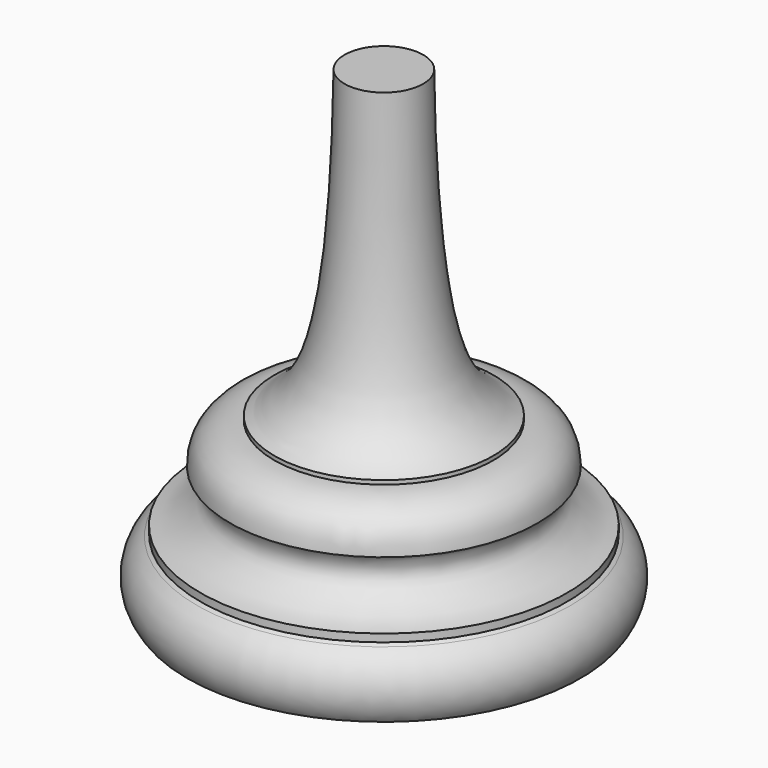
from build123d import *

# Parameters (mm, degrees)
F2_R            = 3
F3_DEPTH        = 1
F3_COPIES_COUNT = 3


# Not quite as in the source:
# - a pattern or mirror of a feature is missing from the dataset's text; its kind, count and spacing are read off the source's solid


with BuildPart() as f1:
    # F0 (on Front) → F1 (revolve)
    with BuildSketch(Plane.XZ):
        with BuildLine():
            ThreePointArc((0, 25), (-7.2712870514, 23.9192053509), (-13.9138726518, 20.7702707693))
            ThreePointArc((-13.9138726518, 20.7702707693), (-16.9329926398, 18.3922201015), (-19.5519464432, 15.5795182943))
            add(Edge.make_bspline(
                [(-23.3200709548, 9.0096776116), (-21.486513797, 9.2002640085), (-17.9330601868, 11.4727622575), (-17.882184425, 13.9799116864), (-18.6395279182, 15.496779924), (-19.5519464432, 15.5795182943)],
                knots=[0, 0, 0, 0, 0.4447205998, 0.7258165522, 1, 1, 1, 1], degree=3))
            Line((-23.3200709548, 9.0096776116), (-23.3200709548, 8.023869816))
            ThreePointArc((-23.3200709548, 8.023869816), (-18.0187025434, 7.9122934085), (-15.399707997, 3.3016726375))
            ThreePointArc((-15.399707997, 3.3016726375), (-15.6915120532, 1.5559363089), (-16.5351986885, 0))
            Line((-16.5351986885, 0), (0, 0))
            Line((0, 0), (0, 25))
        make_face()
        with BuildLine():
            Line((-13.9138726518, 21.280977875), (-13.9138726518, 20.7702707693))
            ThreePointArc((-13.9138726518, 20.7702707693), (-7.2712870514, 23.9192053509), (0, 25))
            Line((0, 25), (0, 60))
            Line((0, 60), (-5, 60))
            add(Edge.make_bspline(
                [(-13.9138726518, 21.280977875), (-13.0526568698, 21.6014376217), (-9.9668374865, 24.3144288022), (-5.488730967, 28.2790772617), (-5, 60)],
                knots=[0, 0, 0, 0, 0.2106788088, 1, 1, 1, 1], degree=3))
        make_face()
        with BuildLine():
            ThreePointArc((-19.5519464432, 15.5795182943), (-16.9329926398, 18.3922201015), (-13.9138726518, 20.7702707693))
            add(Edge.make_bspline(
                [(-19.5519464432, 15.5795182943), (-19.5931974036, 17.273765886), (-18.3786831103, 19.8004802455), (-15.3900210334, 20.7829197498), (-13.9138726518, 20.7702707693)],
                knots=[0, 0, 0, 0, 0.4965371483, 1, 1, 1, 1], degree=3))
        make_face()
        with BuildLine():
            ThreePointArc((-23.3200709548, 8.023869816), (-23.5470299297, 7.8939512806), (-23.7673920649, 7.753133201))
            ThreePointArc((-23.7673920649, 7.753133201), (-24.6899250872, 3.9252514809), (-25, 0))
            Line((-25, 0), (-16.5351986885, 0))
            ThreePointArc((-16.5351986885, 0), (-15.6915120532, 1.5559363089), (-15.399707997, 3.3016726375))
            ThreePointArc((-15.399707997, 3.3016726375), (-18.0187025434, 7.9122934085), (-23.3200709548, 8.023869816))
        make_face()
        with BuildLine():
            ThreePointArc((-25, 0), (-24.6899250872, 3.9252514809), (-23.7673920649, 7.753133201))
            ThreePointArc((-23.7673920649, 7.753133201), (-26.0689127538, 4.1444855759), (-25, 0))
        make_face()
    revolve(axis=Axis((0, 0, 30), (0, 0, 1)))

    # F2 (on face) → F3 (cut)
    with BuildSketch(Plane(origin=(0, 0, 0), x_dir=(1, 0, 0), z_dir=(0, 0, -1))):
        with Locations((19, 0)):
            Circle(F2_R)
    f3 = extrude(amount=-F3_DEPTH, mode=Mode.SUBTRACT)

    # F3_copies: F3 ×3 about axis
    f3_copies_axis = Axis((0, 0, 0), (0, 0, 1))
    for i in range(1, F3_COPIES_COUNT):
        add(f3.rotate(f3_copies_axis, i * 360 / F3_COPIES_COUNT), mode=Mode.SUBTRACT)


solid = f1.part
